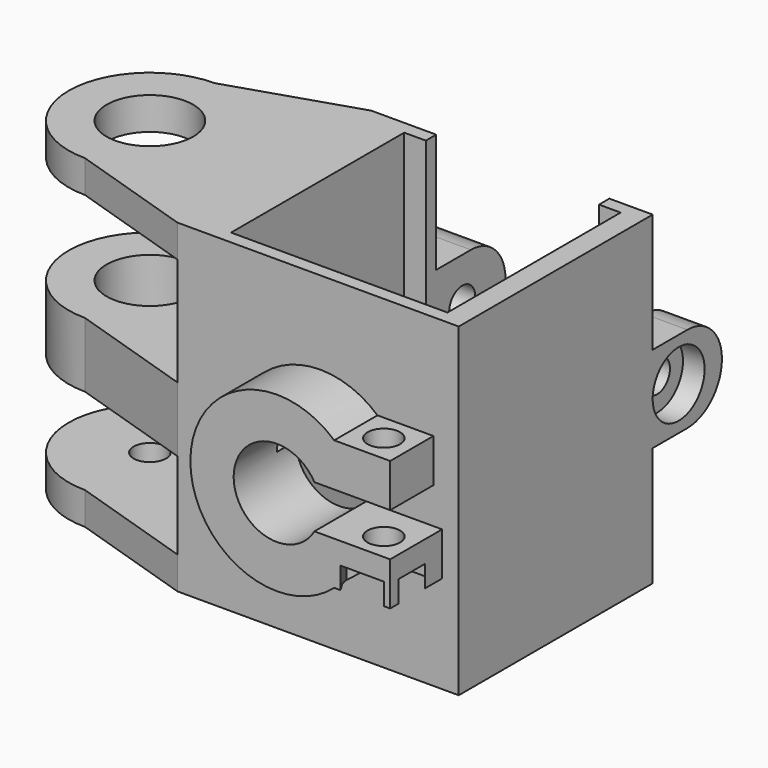
from build123d import *

# Parameters (mm, degrees)
F1_DEPTH  = 30
F3_DEPTH  = 6
F4_DEPTH  = 25
F6_DEPTH  = 15
F7_R      = 1.5
F8_DEPTH  = 25
F9_W      = 4
F9_H      = 8
F9_W_2    = 6
F10_DEPTH = 8
F11_R     = 3.99999
F12_R     = 1.5
F13_DEPTH = 25
F14_START = 27
F0_R      = 1.5
F14_DEPTH = 3
F15_START = 11
F15_DEPTH = 6
F16_DEPTH = 3
F17_R     = 4
F17_R_2   = 1.5
F18_DEPTH = 27
F12_R_2   = 3
F19_DEPTH = 2
F21_DEPTH = 3
F23_START = -2
F22_R     = 1.5
F23_DEPTH = 8


# Not quite as in the source:
# - a fillet or chamfer is up to 0.001 mm smaller than in the source, because OpenCascade refuses the exact size
# - a feature names something its author has since deleted; it is built from what else it names


with BuildPart() as f1:
    # F0 (on Top) → F1 (new body)
    with BuildSketch(Plane.XY):
        Polygon((20, 0), (0, 0), (0, 20), (2, 20), (2, 21.2), (-4, 21.2), (-4, -1.2), (22, -1.2), (22, 21.2), (18, 21.2), (18, 20), (20, 20), align=None)
    extrude(amount=F1_DEPTH)

    # F2 (on face) → F3 (join)
    with BuildSketch(Plane.XZ.offset(1.2)):
        with BuildLine():
            ThreePointArc((6, 15), (8.9647238196, 18.8637033052), (13.4641016151, 17))
            Line((13.4641016151, 17), (17.7459666924, 17))
            ThreePointArc((17.7459666924, 17), (16.8186436725, 19.1840289755), (15.2915026221, 21))
            ThreePointArc((15.2915026221, 21), (6.7084973779, 22.2915026221), (2, 15))
            Line((2, 15), (6, 15))
        make_face()
        with BuildLine():
            ThreePointArc((15.2915026221, 21), (16.8186436725, 19.1840289755), (17.7459666924, 17))
            Line((17.7459666924, 17), (20.4641016151, 17))
            Line((20.4641016151, 17), (20.4641016151, 21))
            Line((20.4641016151, 21), (15.2915026221, 21))
        make_face()
        with BuildLine():
            Line((20.4641016151, 13), (17.7459666924, 13))
            ThreePointArc((17.7459666924, 13), (16.8186436725, 10.8159710245), (15.2915026221, 9))
            Line((15.2915026221, 9), (20.4641016151, 9))
            Line((20.4641016151, 9), (20.4641016151, 13))
        make_face()
        with BuildLine():
            Line((17.7459666924, 13), (13.4641016151, 13))
            ThreePointArc((13.4641016151, 13), (8.9647238196, 11.1362966948), (6, 15))
            Line((6, 15), (2, 15))
            ThreePointArc((2, 15), (6.7084973779, 7.7084973779), (15.2915026221, 9))
            ThreePointArc((15.2915026221, 9), (16.8186436725, 10.8159710245), (17.7459666924, 13))
        make_face()
    extrude(amount=F3_DEPTH)

    # F2 (on face) → F4 (cut)
    with BuildSketch(Plane.XZ.offset(1.2)):
        with BuildLine():
            ThreePointArc((13.4641016151, 13), (13.8637033052, 13.9647238196), (14, 15))
            ThreePointArc((14, 15), (13.8637033052, 16.0352761804), (13.4641016151, 17))
            ThreePointArc((13.4641016151, 17), (8.9647238196, 18.8637033052), (6, 15))
            ThreePointArc((6, 15), (8.9647238196, 11.1362966948), (13.4641016151, 13))
        make_face()
    extrude(amount=-F4_DEPTH, mode=Mode.SUBTRACT)

    # F5 (on face) → F6 (cut)
    with BuildSketch(Plane.XY.offset(30)):
        Polygon((22, -1.2), (3, -1.2), (3, -2.2), (23, -2.2), (23, -1.2), align=None)
    extrude(amount=-F6_DEPTH, mode=Mode.SUBTRACT)

    # F7 (on face) → F8 (cut)
    with BuildSketch(Plane.XY.offset(21)):
        with Locations((17.8778021186, -4.7)):
            Circle(F7_R)
    extrude(amount=-F8_DEPTH, mode=Mode.SUBTRACT)

    # F9 (on face) → F10 (join)
    with BuildSketch(Plane(origin=(0, 21.2, 0), x_dir=(-1, 0, 0), z_dir=(0, 1, 0))):
        with Locations((-20, 15)):
            Rectangle(F9_W, F9_H)
        with Locations((1, 15)):
            Rectangle(F9_W_2, F9_H)
    extrude(amount=F10_DEPTH)

    # F11 (radius 4 in the source; OpenCascade refuses exactly that, so slightly less here)
    f11_edges = [f1.edges().sort_by_distance(p)[0] for p in [
        (20, 29.2, 19),
        (20, 29.2, 11),
        (-1, 29.2, 19),
        (-1, 29.2, 11),
    ]]
    fillet(f11_edges, radius=F11_R)

    # F12 (on face) → F13 (cut)
    with BuildSketch(Plane.YZ.offset(22)):
        with Locations((24.2, 15)):
            Circle(F12_R)
    extrude(amount=-F13_DEPTH, mode=Mode.SUBTRACT)

    # F0 (on Top) → F14 (join)
    with BuildSketch(Plane.XY.offset(F14_START)):
        with BuildLine():
            Line((-4, -1.2), (-4, 21.2))
            Line((-4, 21.2), (-15.5, 17.5))
            ThreePointArc((-15.5, 17.5), (-10.1966991411, 15.3033008589), (-8, 10))
            ThreePointArc((-8, 10), (-10.1966991411, 4.6966991411), (-15.5, 2.5))
            Line((-15.5, 2.5), (-4, -1.2))
        make_face()
        with BuildLine():
            ThreePointArc((-8, 10), (-10.1966991411, 15.3033008589), (-15.5, 17.5))
            ThreePointArc((-15.5, 17.5), (-23, 10), (-15.5, 2.5))
            ThreePointArc((-15.5, 2.5), (-10.1966991411, 4.6966991411), (-8, 10))
        make_face()
        with Locations((-15.5, 10)):
            Circle(F0_R, mode=Mode.SUBTRACT)
        Polygon((20, 0), (0, 0), (0, 20), (2, 20), (2, 21.2), (-4, 21.2), (-4, -1.2), (22, -1.2), (22, 21.2), (18, 21.2), (18, 20), (20, 20), align=None)
    extrude(amount=F14_DEPTH)

    # F0 (on Top) → F15 (join)
    with BuildSketch(Plane.XY.offset(F15_START)):
        with BuildLine():
            ThreePointArc((-8, 10), (-10.1966991411, 15.3033008589), (-15.5, 17.5))
            ThreePointArc((-15.5, 17.5), (-23, 10), (-15.5, 2.5))
            ThreePointArc((-15.5, 2.5), (-10.1966991411, 4.6966991411), (-8, 10))
        make_face()
        with Locations((-15.5, 10)):
            Circle(F0_R, mode=Mode.SUBTRACT)
        with BuildLine():
            Line((-4, -1.2), (-4, 21.2))
            Line((-4, 21.2), (-15.5, 17.5))
            ThreePointArc((-15.5, 17.5), (-10.1966991411, 15.3033008589), (-8, 10))
            ThreePointArc((-8, 10), (-10.1966991411, 4.6966991411), (-15.5, 2.5))
            Line((-15.5, 2.5), (-4, -1.2))
        make_face()
    extrude(amount=F15_DEPTH)

    # F0 (on Top) → F16 (join)
    with BuildSketch(Plane.XY):
        with BuildLine():
            ThreePointArc((-8, 10), (-10.1966991411, 15.3033008589), (-15.5, 17.5))
            ThreePointArc((-15.5, 17.5), (-23, 10), (-15.5, 2.5))
            ThreePointArc((-15.5, 2.5), (-10.1966991411, 4.6966991411), (-8, 10))
        make_face()
        with Locations((-15.5, 10)):
            Circle(F0_R, mode=Mode.SUBTRACT)
        with BuildLine():
            Line((-4, -1.2), (-4, 21.2))
            Line((-4, 21.2), (-15.5, 17.5))
            ThreePointArc((-15.5, 17.5), (-10.1966991411, 15.3033008589), (-8, 10))
            ThreePointArc((-8, 10), (-10.1966991411, 4.6966991411), (-15.5, 2.5))
            Line((-15.5, 2.5), (-4, -1.2))
        make_face()
    extrude(amount=F16_DEPTH)

    # F17 (on face) → F18 (cut)
    with BuildSketch(Plane.XY.offset(30)):
        with Locations((-15.5, 10)):
            Circle(F17_R)
        with Locations((-15.5, 10)):
            Circle(F17_R_2, mode=Mode.SUBTRACT)
    extrude(amount=-F18_DEPTH, mode=Mode.SUBTRACT)

    # F12 (on face) → F19 (cut)
    with BuildSketch(Plane.YZ.offset(22)):
        with Locations((24.2, 15)):
            Circle(F12_R_2)
        with Locations((24.2, 15)):
            Circle(F12_R, mode=Mode.SUBTRACT)
    extrude(amount=-F19_DEPTH, mode=Mode.SUBTRACT)

    # F20 (on face) → F21 (cut)
    with BuildSketch(Plane(origin=(-4, 0, 0), x_dir=(0, -1, 0), z_dir=(-1, 0, 0))):
        Polygon((-21.2, 13.2679491924), (-21.2, 16.7320508076), (-24.2, 18.4641016151), (-27.2, 16.7320508076), (-27.2, 13.2679491924), (-24.2, 11.5358983849), align=None)
    extrude(amount=-F21_DEPTH, mode=Mode.SUBTRACT)

    # F22 (on face) → F23 (cut)
    with BuildSketch(Plane.XY.offset(13).offset(F23_START)):
        Polygon((19.6098529262, -1.7), (16.1457513111, -1.7), (14.4137005035, -4.7), (15.8570761765, -7.2), (19.8985280608, -7.2), (20.4641016151, -6.2203978685), (20.4641016151, -3.1796021315), align=None)
        with Locations((17.8778021186, -4.7)):
            Circle(F22_R, mode=Mode.SUBTRACT)
    extrude(amount=-F23_DEPTH, mode=Mode.SUBTRACT)


solid = f1.part
